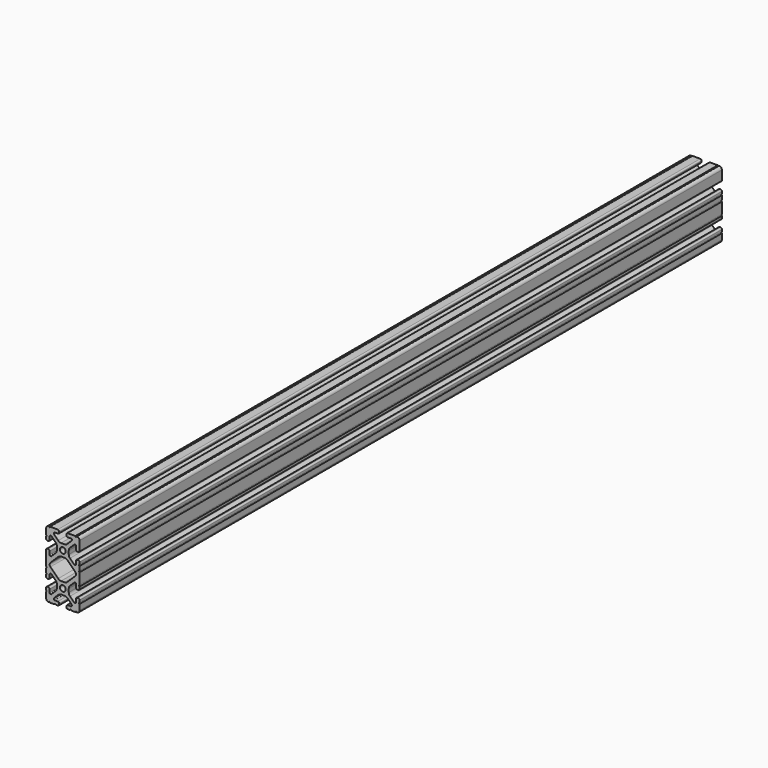
from build123d import *

# Parameters (mm, degrees)
F1_DEPTH = 914.4


# Not quite as in the source:
# - ends of sketch curves that miss each other by under 0.0002 mm in the source are joined


with BuildPart() as f1:
    # F0 (on Front) → F1 (new body)
    with BuildSketch(Plane.XZ):
        with BuildLine():
            ThreePointArc((-88.295226, 46.7995), (-88.8340413673, 46.5763153673), (-89.057226, 46.0375))
            Line((-89.057226, 46.0375), (-88.295226, 46.0375))
            Line((-88.295226, 46.0375), (-88.295226, 46.7995))
        make_face()
        with BuildLine():
            ThreePointArc((-88.295226, 45.2755), (-88.8340413673, 45.4986846327), (-89.057226, 46.0375))
            ThreePointArc((-89.057226, 46.0375), (-88.8340413673, 46.5763153673), (-88.295226, 46.7995))
            Line((-88.295226, 46.7995), (-88.295226, 46.8376))
            Line((-88.295226, 46.8376), (-88.295226, 53.2003))
            ThreePointArc((-88.295226, 53.2003), (-89.057226, 53.9623), (-88.295226, 54.7243))
            Line((-88.295226, 54.7243), (-88.295226, 59.5503))
            ThreePointArc((-88.295226, 59.5503), (-89.057226, 60.3123), (-88.295226, 61.0743))
            Line((-88.295226, 61.0743), (-88.295226, 63.4111))
            ThreePointArc((-88.295226, 63.4111), (-88.756474241, 64.524651759), (-89.870026, 64.9859))
            Line((-89.870026, 64.9859), (-90.784426, 64.9859))
            ThreePointArc((-90.784426, 64.9859), (-91.897977759, 64.524651759), (-92.359226, 63.4111))
            Line((-92.359226, 63.4111), (-92.359226, 59.6519))
            ThreePointArc((-92.359226, 59.6519), (-92.6196080715, 59.0232820715), (-93.248226, 58.7629))
            Line((-93.248226, 58.7629), (-93.816297, 58.7629))
            ThreePointArc((-93.816297, 58.7629), (-94.1565025714, 58.8305710956), (-94.4449149285, 59.0232820715))
            Line((-94.4449149285, 59.0232820715), (-99.1976426, 63.7759964))
            ThreePointArc((-99.1976426, 63.7759964), (-100.2272690035, 65.316943233), (-100.588826, 67.134613))
            Line((-100.588826, 67.134613), (-100.588826, 70.965187))
            ThreePointArc((-100.588826, 70.965187), (-100.2272690035, 72.782856767), (-99.1976417893, 74.3238027893))
            Line((-99.1976417893, 74.3238027893), (-94.4449216, 79.0765246))
            ThreePointArc((-94.4449216, 79.0765246), (-94.1565025714, 79.2692289044), (-93.816297, 79.3369))
            Line((-93.816297, 79.3369), (-93.248226, 79.3369))
            ThreePointArc((-93.248226, 79.3369), (-92.6196080715, 79.0765179285), (-92.359226, 78.4479))
            Line((-92.359226, 78.4479), (-92.359226, 74.6887))
            ThreePointArc((-92.359226, 74.6887), (-91.897977759, 73.575148241), (-90.784426, 73.1139))
            Line((-90.784426, 73.1139), (-89.870026, 73.1139))
            ThreePointArc((-89.870026, 73.1139), (-88.756474241, 73.575148241), (-88.295226, 74.6887))
            Line((-88.295226, 74.6887), (-88.295226, 76.9874))
            Line((-88.295226, 76.9874), (-88.295226, 77.0255))
            ThreePointArc((-88.295226, 77.0255), (-88.8340413673, 77.2486846327), (-89.057226, 77.7875))
            ThreePointArc((-89.057226, 77.7875), (-88.8340413673, 78.3263153673), (-88.295226, 78.5495))
            Line((-88.295226, 78.5495), (-88.295226, 78.5876))
            Line((-88.295226, 78.5876), (-88.295226, 83.3374))
            Line((-88.295226, 83.3374), (-88.295226, 83.3755))
            ThreePointArc((-88.295226, 83.3755), (-88.8340413673, 83.5986846327), (-89.057226, 84.1375))
            ThreePointArc((-89.057226, 84.1375), (-88.8340413673, 84.6763153673), (-88.295226, 84.8995))
            Line((-88.295226, 84.8995), (-88.295226, 84.9376))
            ThreePointArc((-88.295226, 84.9376), (-89.2385712992, 87.1834957351), (-91.4956259934, 88.099899184))
            ThreePointArc((-91.4956259934, 88.099899184), (-92.257626, 87.3379), (-93.019626, 88.0999))
            Line((-93.019626, 88.0999), (-97.807526, 88.0999))
            Line((-97.807526, 88.0999), (-97.845626, 88.0999))
            ThreePointArc((-97.845626, 88.0999), (-98.0688106327, 87.5610846327), (-98.607626, 87.3379))
            ThreePointArc((-98.607626, 87.3379), (-99.1464413673, 87.5610846327), (-99.369626, 88.0999))
            Line((-99.369626, 88.0999), (-99.407726, 88.0999))
            Line((-99.407726, 88.0999), (-101.706426, 88.0999))
            ThreePointArc((-101.706426, 88.0999), (-102.819977759, 87.638651759), (-103.281226, 86.5251))
            Line((-103.281226, 86.5251), (-103.281226, 85.6107))
            ThreePointArc((-103.281226, 85.6107), (-102.819977759, 84.497148241), (-101.706426, 84.0359))
            Line((-101.706426, 84.0359), (-97.947226, 84.0359))
            ThreePointArc((-97.947226, 84.0359), (-97.3186080715, 83.7755179285), (-97.058226, 83.1469))
            Line((-97.058226, 83.1469), (-97.058226, 82.578829))
            ThreePointArc((-97.058226, 82.578829), (-97.1258970956, 82.2386234286), (-97.3186080715, 81.9502110715))
            Line((-97.3186080715, 81.9502110715), (-102.0713224, 77.1974834))
            ThreePointArc((-102.0713224, 77.1974834), (-103.612269233, 76.1678569965), (-105.429939, 75.8063))
            Line((-105.429939, 75.8063), (-109.260513, 75.8063))
            ThreePointArc((-109.260513, 75.8063), (-111.078182767, 76.1678569965), (-112.6191287893, 77.1974842107))
            Line((-112.6191287893, 77.1974842107), (-117.3718506, 81.9502044))
            ThreePointArc((-117.3718506, 81.9502044), (-117.5645549044, 82.2386234286), (-117.632226, 82.578829))
            Line((-117.632226, 82.578829), (-117.632226, 83.1469))
            ThreePointArc((-117.632226, 83.1469), (-117.3718439285, 83.7755179285), (-116.743226, 84.0359))
            Line((-116.743226, 84.0359), (-112.984026, 84.0359))
            ThreePointArc((-112.984026, 84.0359), (-111.870474241, 84.497148241), (-111.409226, 85.6107))
            Line((-111.409226, 85.6107), (-111.409226, 86.5251))
            ThreePointArc((-111.409226, 86.5251), (-111.870474241, 87.638651759), (-112.984026, 88.0999))
            Line((-112.984026, 88.0999), (-115.282726, 88.0999))
            Line((-115.282726, 88.0999), (-115.320826, 88.0999))
            ThreePointArc((-115.320826, 88.0999), (-115.5440106327, 87.5610846327), (-116.082826, 87.3379))
            ThreePointArc((-116.082826, 87.3379), (-116.6216413673, 87.5610846327), (-116.844826, 88.0999))
            Line((-116.844826, 88.0999), (-116.882926, 88.0999))
            Line((-116.882926, 88.0999), (-121.670826, 88.0999))
            ThreePointArc((-121.670826, 88.0999), (-122.432826, 87.3379), (-123.194826, 88.0999))
            ThreePointArc((-123.194826, 88.0999), (-125.4518807008, 87.1834957351), (-126.3953026035, 84.937600304))
            Line((-126.3953026035, 84.937600304), (-126.395226, 84.8995000033))
            ThreePointArc((-126.395226, 84.8995000033), (-125.8564106327, 84.6763153673), (-125.633226, 84.1375))
            ThreePointArc((-125.633226, 84.1375), (-125.8564106327, 83.5986846327), (-126.395226, 83.3755))
            Line((-126.395226, 83.3755), (-126.395226, 83.3374))
            Line((-126.395226, 83.3374), (-126.395226, 78.5495))
            ThreePointArc((-126.395226, 78.5495), (-125.633226, 77.7875), (-126.395226, 77.0255))
            Line((-126.395226, 77.0255), (-126.395226, 74.6887))
            ThreePointArc((-126.395226, 74.6887), (-125.933977759, 73.575148241), (-124.820426, 73.1139))
            Line((-124.820426, 73.1139), (-123.906026, 73.1139))
            ThreePointArc((-123.906026, 73.1139), (-122.792474241, 73.575148241), (-122.331226, 74.6887))
            Line((-122.331226, 74.6887), (-122.331226, 78.4479))
            ThreePointArc((-122.331226, 78.4479), (-122.0708439285, 79.0765179285), (-121.442226, 79.3369))
            Line((-121.442226, 79.3369), (-120.874155, 79.3369))
            ThreePointArc((-120.874155, 79.3369), (-120.5339494286, 79.2692289044), (-120.2455370715, 79.0765179285))
            Line((-120.2455370715, 79.0765179285), (-115.4928094, 74.3238036))
            ThreePointArc((-115.4928094, 74.3238036), (-114.4631829965, 72.782856767), (-114.101626, 70.965187))
            Line((-114.101626, 70.965187), (-114.101626, 67.134613))
            ThreePointArc((-114.101626, 67.134613), (-114.4631829965, 65.316943233), (-115.4928102107, 63.7759972107))
            Line((-115.4928102107, 63.7759972107), (-120.2455304, 59.0232754))
            ThreePointArc((-120.2455304, 59.0232754), (-120.5339494286, 58.8305710956), (-120.874155, 58.7629))
            Line((-120.874155, 58.7629), (-121.442226, 58.7629))
            ThreePointArc((-121.442226, 58.7629), (-122.0708439285, 59.0232820715), (-122.331226, 59.6519))
            Line((-122.331226, 59.6519), (-122.331226, 63.4111))
            ThreePointArc((-122.331226, 63.4111), (-122.792474241, 64.524651759), (-123.906026, 64.9859))
            Line((-123.906026, 64.9859), (-124.820426, 64.9859))
            ThreePointArc((-124.820426, 64.9859), (-125.933977759, 64.524651759), (-126.395226, 63.4111))
            Line((-126.395226, 63.4111), (-126.395226, 61.1124))
            Line((-126.395226, 61.1124), (-126.395226, 61.0743))
            ThreePointArc((-126.395226, 61.0743), (-125.8564106327, 60.8511153673), (-125.633226, 60.3123))
            ThreePointArc((-125.633226, 60.3123), (-125.8564106327, 59.7734846327), (-126.395226, 59.5503))
            Line((-126.395226, 59.5503), (-126.395226, 59.5122))
            Line((-126.395226, 59.5122), (-126.395226, 54.7624))
            Line((-126.395226, 54.7624), (-126.395226, 54.7243))
            ThreePointArc((-126.395226, 54.7243), (-125.8564106327, 54.5011153673), (-125.633226, 53.9623))
            ThreePointArc((-125.633226, 53.9623), (-125.8564106327, 53.4234846327), (-126.395226, 53.2003))
            Line((-126.395226, 53.2003), (-126.395226, 53.1622))
            Line((-126.395226, 53.1622), (-126.395226, 46.7995))
            ThreePointArc((-126.395226, 46.7995), (-125.633226, 46.0375), (-126.395226, 45.2755))
            Line((-126.395226, 45.2755), (-126.395226, 40.4495))
            ThreePointArc((-126.395226, 40.4495), (-125.633226, 39.6875), (-126.395226, 38.9255))
            Line((-126.395226, 38.9255), (-126.395226, 36.5887))
            ThreePointArc((-126.395226, 36.5887), (-125.933977759, 35.475148241), (-124.820426, 35.0139))
            Line((-124.820426, 35.0139), (-123.906026, 35.0139))
            ThreePointArc((-123.906026, 35.0139), (-122.792474241, 35.475148241), (-122.331226, 36.5887))
            Line((-122.331226, 36.5887), (-122.331226, 40.3479))
            ThreePointArc((-122.331226, 40.3479), (-122.0708439285, 40.9765179285), (-121.442226, 41.2369))
            Line((-121.442226, 41.2369), (-120.874155, 41.2369))
            ThreePointArc((-120.874155, 41.2369), (-120.5339494286, 41.1692289044), (-120.2455370715, 40.9765179285))
            Line((-120.2455370715, 40.9765179285), (-115.4928094, 36.2238036))
            ThreePointArc((-115.4928094, 36.2238036), (-114.4631829965, 34.682856767), (-114.101626, 32.865187))
            Line((-114.101626, 32.865187), (-114.101626, 29.034613))
            ThreePointArc((-114.101626, 29.034613), (-114.4631829965, 27.216943233), (-115.4928102107, 25.6759972107))
            Line((-115.4928102107, 25.6759972107), (-120.2455304, 20.9232754))
            ThreePointArc((-120.2455304, 20.9232754), (-120.5339494286, 20.7305710956), (-120.874155, 20.6629))
            Line((-120.874155, 20.6629), (-121.442226, 20.6629))
            ThreePointArc((-121.442226, 20.6629), (-122.0708439285, 20.9232820715), (-122.331226, 21.5519))
            Line((-122.331226, 21.5519), (-122.331226, 25.3111))
            ThreePointArc((-122.331226, 25.3111), (-122.792474241, 26.424651759), (-123.906026, 26.8859))
            Line((-123.906026, 26.8859), (-124.820426, 26.8859))
            ThreePointArc((-124.820426, 26.8859), (-125.933977759, 26.424651759), (-126.395226, 25.3111))
            Line((-126.395226, 25.3111), (-126.395226, 22.9743))
            ThreePointArc((-126.395226, 22.9743), (-125.633226, 22.2123), (-126.395226, 21.4503))
            Line((-126.395226, 21.4503), (-126.395226, 16.6624))
            Line((-126.395226, 16.6624), (-126.395226, 16.6243))
            ThreePointArc((-126.395226, 16.6243), (-125.8564106327, 16.4011153673), (-125.633226, 15.8623))
            ThreePointArc((-125.633226, 15.8623), (-125.8564106327, 15.3234846327), (-126.395226, 15.1003))
            Line((-126.395226, 15.1003), (-126.395226, 15.0622))
            ThreePointArc((-126.395226, 15.0622), (-125.4518807008, 12.8163042649), (-123.1948260066, 11.899900816))
            ThreePointArc((-123.1948260066, 11.899900816), (-122.432826, 12.6619), (-121.670826, 11.8999))
            Line((-121.670826, 11.8999), (-116.844826, 11.8999))
            ThreePointArc((-116.844826, 11.8999), (-116.082826, 12.6619), (-115.320826, 11.8999))
            Line((-115.320826, 11.8999), (-112.984026, 11.8999))
            ThreePointArc((-112.984026, 11.8999), (-111.870474241, 12.361148241), (-111.409226, 13.4747))
            Line((-111.409226, 13.4747), (-111.409226, 14.3891))
            ThreePointArc((-111.409226, 14.3891), (-111.870474241, 15.502651759), (-112.984026, 15.9639))
            Line((-112.984026, 15.9639), (-116.743226, 15.9639))
            ThreePointArc((-116.743226, 15.9639), (-117.3718439285, 16.2242820715), (-117.632226, 16.8529))
            Line((-117.632226, 16.8529), (-117.632226, 17.420971))
            ThreePointArc((-117.632226, 17.420971), (-117.5645549044, 17.7611765714), (-117.3718439285, 18.0495889285))
            Line((-117.3718439285, 18.0495889285), (-112.6191296, 22.8023166))
            ThreePointArc((-112.6191296, 22.8023166), (-111.078182767, 23.8319430035), (-109.260513, 24.1935))
            Line((-109.260513, 24.1935), (-105.429939, 24.1935))
            ThreePointArc((-105.429939, 24.1935), (-103.612269233, 23.8319430035), (-102.0713232107, 22.8023157893))
            Line((-102.0713232107, 22.8023157893), (-97.3186014, 18.0495956))
            ThreePointArc((-97.3186014, 18.0495956), (-97.1258970956, 17.7611765714), (-97.058226, 17.420971))
            Line((-97.058226, 17.420971), (-97.058226, 16.8529))
            ThreePointArc((-97.058226, 16.8529), (-97.3186080715, 16.2242820715), (-97.947226, 15.9639))
            Line((-97.947226, 15.9639), (-101.706426, 15.9639))
            ThreePointArc((-101.706426, 15.9639), (-102.819977759, 15.502651759), (-103.281226, 14.3891))
            Line((-103.281226, 14.3891), (-103.281226, 13.4747))
            ThreePointArc((-103.281226, 13.4747), (-102.819977759, 12.361148241), (-101.706426, 11.8999))
            Line((-101.706426, 11.8999), (-99.369626, 11.8999))
            ThreePointArc((-99.369626, 11.8999), (-98.607626, 12.6619), (-97.845626, 11.8999))
            Line((-97.845626, 11.8999), (-93.019626, 11.8999))
            ThreePointArc((-93.019626, 11.8999), (-92.257626, 12.6619), (-91.495626, 11.8999))
            ThreePointArc((-91.495626, 11.8999), (-89.2385712992, 12.8163042649), (-88.2951493965, 15.062199696))
            Line((-88.2951493965, 15.062199696), (-88.295226, 15.1002999967))
            ThreePointArc((-88.295226, 15.1002999967), (-88.8340413673, 15.3234846327), (-89.057226, 15.8623))
            ThreePointArc((-89.057226, 15.8623), (-88.8340413673, 16.4011153673), (-88.295226, 16.6243))
            Line((-88.295226, 16.6243), (-88.295226, 16.6624))
            Line((-88.295226, 16.6624), (-88.295226, 21.4503))
            ThreePointArc((-88.295226, 21.4503), (-89.057226, 22.2123), (-88.295226, 22.9743))
            Line((-88.295226, 22.9743), (-88.295226, 25.3111))
            ThreePointArc((-88.295226, 25.3111), (-88.756474241, 26.424651759), (-89.870026, 26.8859))
            Line((-89.870026, 26.8859), (-90.784426, 26.8859))
            ThreePointArc((-90.784426, 26.8859), (-91.897977759, 26.424651759), (-92.359226, 25.3111))
            Line((-92.359226, 25.3111), (-92.359226, 21.5519))
            ThreePointArc((-92.359226, 21.5519), (-92.6196080715, 20.9232820715), (-93.248226, 20.6629))
            Line((-93.248226, 20.6629), (-93.816297, 20.6629))
            ThreePointArc((-93.816297, 20.6629), (-94.1565025714, 20.7305710956), (-94.4449149285, 20.9232820715))
            Line((-94.4449149285, 20.9232820715), (-99.1976426, 25.6759964))
            ThreePointArc((-99.1976426, 25.6759964), (-100.2272690035, 27.216943233), (-100.588826, 29.034613))
            Line((-100.588826, 29.034613), (-100.588826, 32.865187))
            ThreePointArc((-100.588826, 32.865187), (-100.2272690035, 34.682856767), (-99.1976417893, 36.2238027893))
            Line((-99.1976417893, 36.2238027893), (-94.4449216, 40.9765246))
            ThreePointArc((-94.4449216, 40.9765246), (-94.1565025714, 41.1692289044), (-93.816297, 41.2369))
            Line((-93.816297, 41.2369), (-93.248226, 41.2369))
            ThreePointArc((-93.248226, 41.2369), (-92.6196080715, 40.9765179285), (-92.359226, 40.3479))
            Line((-92.359226, 40.3479), (-92.359226, 36.5887))
            ThreePointArc((-92.359226, 36.5887), (-91.897977759, 35.475148241), (-90.784426, 35.0139))
            Line((-90.784426, 35.0139), (-89.870026, 35.0139))
            ThreePointArc((-89.870026, 35.0139), (-88.756474241, 35.475148241), (-88.295226, 36.5887))
            Line((-88.295226, 36.5887), (-88.295226, 38.9255))
            ThreePointArc((-88.295226, 38.9255), (-89.057226, 39.6875), (-88.295226, 40.4495))
            Line((-88.295226, 40.4495), (-88.295226, 45.2374))
            Line((-88.295226, 45.2374), (-88.295226, 45.2755))
        make_face()
        with BuildLine():
            ThreePointArc((-112.6191287893, 60.9023157893), (-111.078182767, 61.9319430035), (-109.260513, 62.2935))
            Line((-109.260513, 62.2935), (-105.429939, 62.2935))
            ThreePointArc((-105.429939, 62.2935), (-103.612269233, 61.9319430035), (-102.0713232107, 60.9023157893))
            Line((-102.0713232107, 60.9023157893), (-93.2343576, 52.0653518))
            ThreePointArc((-93.2343576, 52.0653518), (-92.3788348, 49.9999), (-93.2343631922, 47.9344537922))
            Line((-93.2343631922, 47.9344537922), (-102.0713224, 39.0974834))
            ThreePointArc((-102.0713224, 39.0974834), (-103.612269233, 38.0678569965), (-105.429939, 37.7063))
            Line((-105.429939, 37.7063), (-109.260513, 37.7063))
            ThreePointArc((-109.260513, 37.7063), (-111.078182767, 38.0678569965), (-112.6191287893, 39.0974842107))
            Line((-112.6191287893, 39.0974842107), (-121.4560944, 47.9344482))
            ThreePointArc((-121.4560944, 47.9344482), (-122.3116172, 49.9999), (-121.4560888078, 52.0653462078))
            Line((-121.4560888078, 52.0653462078), (-112.6191287893, 60.9023157893))
        make_face(mode=Mode.SUBTRACT)
        with BuildLine():
            ThreePointArc((-107.345226, 27.6225), (-109.6980531037, 28.5970728963), (-110.672626, 30.9499))
            ThreePointArc((-110.672626, 30.9499), (-109.6980531037, 33.3027271037), (-107.345226, 34.2773))
            ThreePointArc((-107.345226, 34.2773), (-104.9923988963, 33.3027271037), (-104.017826, 30.9499))
            ThreePointArc((-104.017826, 30.9499), (-104.9923988963, 28.5970728963), (-107.345226, 27.6225))
        make_face(mode=Mode.SUBTRACT)
        with BuildLine():
            ThreePointArc((-107.345226, 65.7225), (-109.6980531037, 66.6970728963), (-110.672626, 69.0499))
            ThreePointArc((-110.672626, 69.0499), (-109.6980531037, 71.4027271037), (-107.345226, 72.3773))
            ThreePointArc((-107.345226, 72.3773), (-104.9923988963, 71.4027271037), (-104.017826, 69.0499))
            ThreePointArc((-104.017826, 69.0499), (-104.9923988963, 66.6970728963), (-107.345226, 65.7225))
        make_face(mode=Mode.SUBTRACT)
        with BuildLine():
            Line((-88.295226, 46.0375), (-89.057226, 46.0375))
            ThreePointArc((-89.057226, 46.0375), (-88.8340413673, 45.4986846327), (-88.295226, 45.2755))
            Line((-88.295226, 45.2755), (-88.295226, 46.0375))
        make_face()
        with BuildLine():
            ThreePointArc((-89.057226, 77.7875), (-88.8340413673, 77.2486846327), (-88.295226, 77.0255))
            Line((-88.295226, 77.0255), (-88.295226, 77.7875))
            Line((-88.295226, 77.7875), (-89.057226, 77.7875))
        make_face()
        with BuildLine():
            Line((-88.295226, 15.8623), (-88.295226, 16.6243))
            ThreePointArc((-88.295226, 16.6243), (-88.8340413673, 16.4011153673), (-89.057226, 15.8623))
            Line((-89.057226, 15.8623), (-88.295226, 15.8623))
        make_face()
        with BuildLine():
            Line((-89.057226, 77.7875), (-88.295226, 77.7875))
            Line((-88.295226, 77.7875), (-88.295226, 78.5495))
            ThreePointArc((-88.295226, 78.5495), (-88.8340413673, 78.3263153673), (-89.057226, 77.7875))
        make_face()
        with BuildLine():
            Line((-88.295226, 15.1002999967), (-88.295226, 15.8623))
            Line((-88.295226, 15.8623), (-89.057226, 15.8623))
            ThreePointArc((-89.057226, 15.8623), (-88.8340413673, 15.3234846327), (-88.295226, 15.1003))
        make_face()
        with BuildLine():
            ThreePointArc((-89.057226, 84.1375), (-88.8340413673, 83.5986846327), (-88.295226, 83.3755))
            Line((-88.295226, 83.3755), (-88.295226, 84.1375))
            Line((-88.295226, 84.1375), (-89.057226, 84.1375))
        make_face()
        with BuildLine():
            Line((-89.057226, 84.1375), (-88.295226, 84.1375))
            Line((-88.295226, 84.1375), (-88.295226, 84.8995000033))
            ThreePointArc((-88.295226, 84.8995), (-88.8340413673, 84.6763153673), (-89.057226, 84.1375))
        make_face()
        with BuildLine():
            ThreePointArc((-98.607626, 87.3379), (-98.0688106327, 87.5610846327), (-97.845626, 88.0999))
            Line((-97.845626, 88.0999), (-98.607626, 88.0999))
            Line((-98.607626, 88.0999), (-98.607626, 87.3379))
        make_face()
        with BuildLine():
            Line((-98.607626, 87.3379), (-98.607626, 88.0999))
            Line((-98.607626, 88.0999), (-99.369626, 88.0999))
            ThreePointArc((-99.369626, 88.0999), (-99.1464413673, 87.5610846327), (-98.607626, 87.3379))
        make_face()
        with BuildLine():
            Line((-126.395226, 15.8623), (-126.395226, 15.1002999967))
            ThreePointArc((-126.395226, 15.1003), (-125.8564106327, 15.3234846327), (-125.633226, 15.8623))
            Line((-125.633226, 15.8623), (-126.395226, 15.8623))
        make_face()
        with BuildLine():
            Line((-126.395226, 16.6243), (-126.395226, 15.8623))
            Line((-126.395226, 15.8623), (-125.633226, 15.8623))
            ThreePointArc((-125.633226, 15.8623), (-125.8564106327, 16.4011153673), (-126.395226, 16.6243))
        make_face()
        with BuildLine():
            ThreePointArc((-116.082826, 87.3379), (-115.5440106327, 87.5610846327), (-115.320826, 88.0999))
            Line((-115.320826, 88.0999), (-116.082826, 88.0999))
            Line((-116.082826, 88.0999), (-116.082826, 87.3379))
        make_face()
        with BuildLine():
            Line((-116.082826, 87.3379), (-116.082826, 88.0999))
            Line((-116.082826, 88.0999), (-116.844826, 88.0999))
            ThreePointArc((-116.844826, 88.0999), (-116.6216413673, 87.5610846327), (-116.082826, 87.3379))
        make_face()
        with BuildLine():
            ThreePointArc((-125.633226, 84.1375), (-125.8564106327, 84.6763153673), (-126.395226, 84.8995))
            Line((-126.395226, 84.8995000033), (-126.395226, 84.1375))
            Line((-126.395226, 84.1375), (-125.633226, 84.1375))
        make_face()
        with BuildLine():
            Line((-125.633226, 84.1375), (-126.395226, 84.1375))
            Line((-126.395226, 84.1375), (-126.395226, 83.3755))
            ThreePointArc((-126.395226, 83.3755), (-125.8564106327, 83.5986846327), (-125.633226, 84.1375))
        make_face()
        with BuildLine():
            Line((-126.395226, 53.9623), (-126.395226, 53.2003))
            ThreePointArc((-126.395226, 53.2003), (-125.8564106327, 53.4234846327), (-125.633226, 53.9623))
            Line((-125.633226, 53.9623), (-126.395226, 53.9623))
        make_face()
        with BuildLine():
            Line((-126.395226, 54.7243), (-126.395226, 53.9623))
            Line((-126.395226, 53.9623), (-125.633226, 53.9623))
            ThreePointArc((-125.633226, 53.9623), (-125.8564106327, 54.5011153673), (-126.395226, 54.7243))
        make_face()
        with BuildLine():
            Line((-126.395226, 60.3123), (-126.395226, 59.5503))
            ThreePointArc((-126.395226, 59.5503), (-125.8564106327, 59.7734846327), (-125.633226, 60.3123))
            Line((-125.633226, 60.3123), (-126.395226, 60.3123))
        make_face()
        with BuildLine():
            Line((-126.395226, 61.0743), (-126.395226, 60.3123))
            Line((-126.395226, 60.3123), (-125.633226, 60.3123))
            ThreePointArc((-125.633226, 60.3123), (-125.8564106327, 60.8511153673), (-126.395226, 61.0743))
        make_face()
    extrude(amount=-F1_DEPTH)


solid = f1.part
